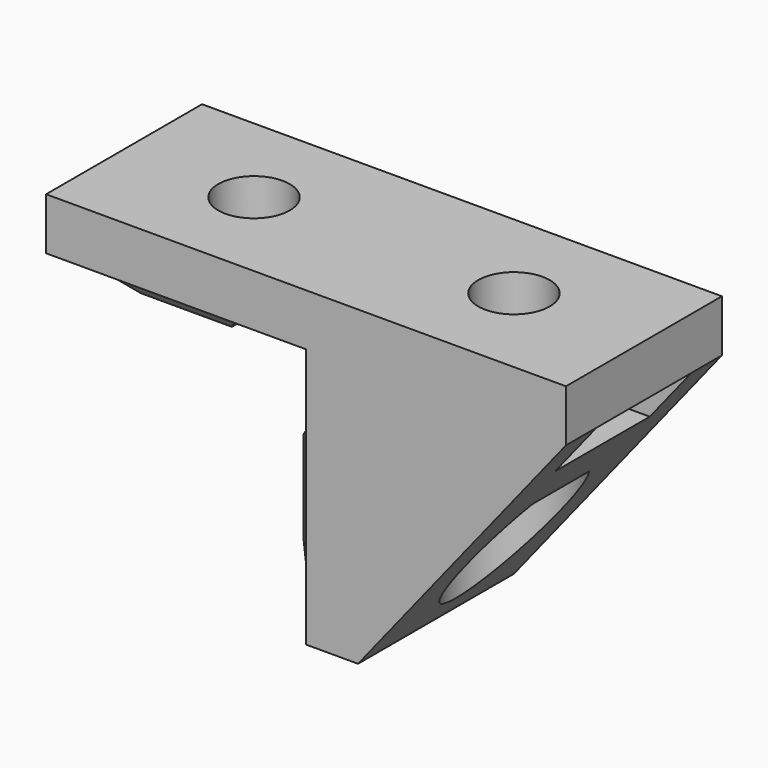
from build123d import *

# Parameters (mm, degrees)
F0_W      = 40
F0_H      = 15
F1_DEPTH  = 4
F2_W      = 9
F2_H      = 15
F2_W_2    = 4
F3_DEPTH  = 1
F4_DEPTH  = 19
F5_W      = 15
F5_H      = 9
F6_DEPTH  = 1
F7_SIZE   = 0.99999
F9_DEPTH  = 15
F12_DEPTH = 4
F13_R     = 2.75
F14_DEPTH = 24.001
F15_R     = 4.5
F16_DEPTH = 12


# Not quite as in the source:
# - a fillet or chamfer is up to 0.001 mm smaller than in the source, because OpenCascade refuses the exact size


with BuildPart() as f1:
    # F0 (on Top) → F1 (new body)
    with BuildSketch(Plane.XY):
        with Locations((20, 7.5)):
            Rectangle(F0_W, F0_H)
    extrude(amount=F1_DEPTH)

    # F2 (on face) → F3 (join)
    with BuildSketch(Plane(origin=(0, 0, 0), x_dir=(1, 0, 0), z_dir=(0, 0, -1))):
        with Locations((10, -7.5)):
            Rectangle(F2_W, F2_H)
        with Locations((22, -7.5)):
            Rectangle(F2_W_2, F2_H)
    extrude(amount=F3_DEPTH)

    # F4 (add): a face of the model
    f4_faces = [f1.faces().sort_by_distance(p)[0] for p in [
        (22, 7.5, -1),
    ]]
    extrude(f4_faces, amount=F4_DEPTH)

    # F5 (on face) → F6 (join)
    with BuildSketch(Plane(origin=(20, 0, 0), x_dir=(0, -1, 0), z_dir=(-1, 0, 0))):
        with Locations((-7.5, -10)):
            Rectangle(F5_W, F5_H)
    extrude(amount=F6_DEPTH)

    # F7 (size 1 in the source; OpenCascade refuses exactly that, so slightly less here)
    f7_edges = [f1.edges().sort_by_distance(p)[0] for p in [
        (19, 15, -10),
        (19, 7.5, -14.5),
        (19, 0, -10),
        (19, 7.5, -5.5),
        (10, 0, -1),
        (5.5, 7.5, -1),
        (10, 15, -1),
        (14.5, 7.5, -1),
    ]]
    chamfer(f7_edges, length=F7_SIZE)

    # F8 (on face) → F9 (join, through all)
    with BuildSketch(Plane.XZ):
        Polygon((40, 0), (24, 0), (24, -20), align=None)
    extrude(amount=-F9_DEPTH)

    # F11 (on offset) → F12 (cut)
    with BuildSketch(Plane.XY):
        Polygon((26.05, 5.2194664367), (30, 2.9389328734), (40, 2.9389328734), (40, 12.0610671266), (30, 12.0610671266), (26.05, 9.7805335633), align=None)
    extrude(amount=-F12_DEPTH, mode=Mode.SUBTRACT)

    # F13 (on face) → F14 (cut, through all)
    with BuildSketch(Plane.XY.offset(4)):
        with Locations((30, 7.5)):
            Circle(F13_R)
        with Locations((10, 7.5)):
            Circle(F13_R)
    extrude(amount=-F14_DEPTH, mode=Mode.SUBTRACT)

    # F15 (on face) → F16 (cut)
    with BuildSketch(Plane(origin=(0, 0, -20), x_dir=(1, 0, 0), z_dir=(0, 0, -1))):
        with Locations((30, -7.5)):
            Circle(F15_R)
    extrude(amount=-F16_DEPTH, mode=Mode.SUBTRACT)


solid = f1.part
